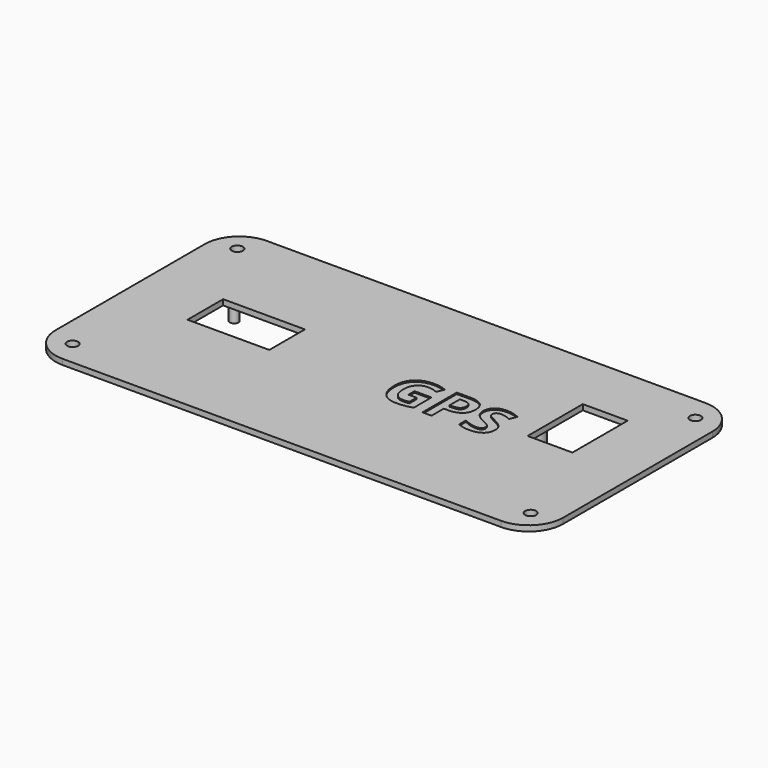
from build123d import *

# Parameters (mm, degrees)
F1_DEPTH      = 3.5
F0_W          = 147.1034944444
F0_H          = 74
F2_DEPTH      = 1.6
F3_W          = 23.7
F3_H          = 12.9
F3_W_2        = 13
F3_H_2        = 20
F4_DEPTH      = 1.601
F3_R          = 1.25
F5_DEPTH      = 5
F3_R_2        = 2.5
F6_DEPTH      = 11
F7_R          = 10
F8_R          = 1.25
F9_DEPTH      = 8
F10_R         = 1.25
F11_DEPTH     = 8
F12_R         = 1.25
F13_DEPTH     = 8
F14_R         = 1.25
F15_DEPTH     = 8
F16_R         = 1.6
F17_DEPTH     = 12.601
F19_TEXT_SIZE = 17.4003174632
F20_DEPTH     = 0.4


# Not quite as in the source:
# - Text() gives the source's letters only with a copy of the font that has no kerning and outlines rounded to 1/6400 em; it was checked with that copy


with BuildPart() as f1:
    # F0 (on Top) → F1 (new body)
    with BuildSketch(Plane.XY):
        with BuildLine():
            Line((62, 27), (-62, 27))
            Line((-62, 27), (-62, -27))
            Line((-62, -27), (62, -27))
            ThreePointArc((62, -27), (65.1034944444, 0), (62, 27))
        make_face()
        with BuildLine():
            ThreePointArc((60.7228645351, 25.4), (63.5034944444, 0), (60.7228645351, -25.4))
            Line((60.7228645351, -25.4), (-60.4, -25.4))
            Line((-60.4, -25.4), (-60.4, 25.4))
            Line((-60.4, 25.4), (60.7228645351, 25.4))
        make_face(mode=Mode.SUBTRACT)
    extrude(amount=-F1_DEPTH)


with BuildPart() as f2:
    # F0 (on Top) → F2 (new body)
    with BuildSketch(Plane.XY):
        with Locations((1.5517472222, 0)):
            Rectangle(F0_W, F0_H)
        with BuildLine():
            Line((-62, -27), (-62, 27))
            Line((-62, 27), (62, 27))
            ThreePointArc((62, 27), (65.1034944444, 0), (62, -27))
            Line((62, -27), (-62, -27))
        make_face(mode=Mode.SUBTRACT)
        with BuildLine():
            Line((62, 27), (-62, 27))
            Line((-62, 27), (-62, -27))
            Line((-62, -27), (62, -27))
            ThreePointArc((62, -27), (65.1034944444, 0), (62, 27))
        make_face()
        with BuildLine():
            ThreePointArc((60.7228645351, 25.4), (63.5034944444, 0), (60.7228645351, -25.4))
            Line((60.7228645351, -25.4), (-60.4, -25.4))
            Line((-60.4, -25.4), (-60.4, 25.4))
            Line((-60.4, 25.4), (60.7228645351, 25.4))
        make_face(mode=Mode.SUBTRACT)
        with BuildLine():
            Line((-60.4, -25.4), (60.7228645351, -25.4))
            ThreePointArc((60.7228645351, -25.4), (63.5034944444, 0), (60.7228645351, 25.4))
            Line((60.7228645351, 25.4), (-60.4, 25.4))
            Line((-60.4, 25.4), (-60.4, -25.4))
        make_face()
    extrude(amount=F2_DEPTH)

    # F3 (on face) → F4 (cut, through all)
    with BuildSketch(Plane.XY):
        with Locations((-40.0405414402, 2.075)):
            Rectangle(F3_W, F3_H)
        with Locations((50.30156672, 9.2107076198)):
            Rectangle(F3_W_2, F3_H_2)
    extrude(amount=F4_DEPTH, mode=Mode.SUBTRACT)

    # F7
    f7_edges = [f2.edges().sort_by_distance(p)[0] for p in [
        (75.103494, 37, 0.8),
        (-72, 37, 0.8),
        (-72, -37, 0.8),
        (75.103494, -37, 0.8),
    ]]
    fillet(f7_edges, radius=F7_R)

    # F16 (on face) → F17 (cut, through all)
    with BuildSketch(Plane.XY.offset(1.6)):
        with Locations((-64.8284271247, 29.8284271247)):
            Circle(F16_R)
        with Locations((67.9319215691, 29.8284271247)):
            Circle(F16_R)
        with Locations((-64.8284271247, -29.8284271247)):
            Circle(F16_R)
        with Locations((67.9319215691, -29.8284271247)):
            Circle(F16_R)
    extrude(amount=-F17_DEPTH, mode=Mode.SUBTRACT)

    # F19 (on face) → F20 (cut)
    with BuildSketch(Plane.XY.offset(1.6)):
        with Locations((3.818041645, -6.6011277959)):
            Text('GPS', F19_TEXT_SIZE, font='Open Sans', font_style=FontStyle.BOLD, text_align=(TextAlign.LEFT, TextAlign.BOTTOM))
    extrude(amount=-F20_DEPTH, mode=Mode.SUBTRACT)


with BuildPart() as f5:
    # F3 (on face) → F5 (new body)
    with BuildSketch(Plane.XY):
        with Locations((-51.1905414402, -11.65)):
            Circle(F3_R)
    extrude(amount=-F5_DEPTH)


with BuildPart() as f5b:
    # F3 (on face) → F5, piece 2 (new body)
    with BuildSketch(Plane.XY):
        with Locations((-28.8905414402, -11.65)):
            Circle(F3_R)
    extrude(amount=-F5_DEPTH)


with BuildPart() as f5c:
    # F3 (on face) → F5, piece 3 (new body)
    with BuildSketch(Plane.XY):
        with Locations((-28.8905414402, 11.65)):
            Circle(F3_R)
    extrude(amount=-F5_DEPTH)


with BuildPart() as f5d:
    # F3 (on face) → F5, piece 4 (new body)
    with BuildSketch(Plane.XY):
        with Locations((-51.1905414402, 11.65)):
            Circle(F3_R)
    extrude(amount=-F5_DEPTH)


with BuildPart() as f6:
    # F3 (on face) → F6 (new body)
    with BuildSketch(Plane.XY):
        with Locations((12.470341146, 15.25)):
            Circle(F3_R_2)
    extrude(amount=-F6_DEPTH)

    # F12 (on face) → F13 (cut)
    with BuildSketch(Plane(origin=(0, 0, -11), x_dir=(1, 0, 0), z_dir=(0, 0, -1))):
        with Locations((12.470341146, -15.25)):
            Circle(F12_R)
    extrude(amount=-F13_DEPTH, mode=Mode.SUBTRACT)


with BuildPart() as f6b:
    # F3 (on face) → F6, piece 2 (new body)
    with BuildSketch(Plane.XY):
        with Locations((33.470341146, 15.25)):
            Circle(F3_R_2)
    extrude(amount=-F6_DEPTH)

    # F14 (on face) → F15 (cut)
    with BuildSketch(Plane(origin=(0, 0, -11), x_dir=(1, 0, 0), z_dir=(0, 0, -1))):
        with Locations((33.470341146, -15.25)):
            Circle(F14_R)
    extrude(amount=-F15_DEPTH, mode=Mode.SUBTRACT)


with BuildPart() as f6c:
    # F3 (on face) → F6, piece 3 (new body)
    with BuildSketch(Plane.XY):
        with Locations((33.470341146, -15.25)):
            Circle(F3_R_2)
    extrude(amount=-F6_DEPTH)

    # F10 (on face) → F11 (cut)
    with BuildSketch(Plane(origin=(0, 0, -11), x_dir=(1, 0, 0), z_dir=(0, 0, -1))):
        with Locations((33.470341146, 15.25)):
            Circle(F10_R)
    extrude(amount=-F11_DEPTH, mode=Mode.SUBTRACT)


with BuildPart() as f6d:
    # F3 (on face) → F6, piece 4 (new body)
    with BuildSketch(Plane.XY):
        with Locations((12.470341146, -15.25)):
            Circle(F3_R_2)
    extrude(amount=-F6_DEPTH)

    # F8 (on face) → F9 (cut)
    with BuildSketch(Plane(origin=(0, 0, -11), x_dir=(1, 0, 0), z_dir=(0, 0, -1))):
        with Locations((12.470341146, 15.25)):
            Circle(F8_R)
    extrude(amount=-F9_DEPTH, mode=Mode.SUBTRACT)


solid = Compound([f1.part, f2.part, f5.part, f5b.part, f5c.part, f5d.part, f6.part, f6b.part, f6c.part, f6d.part])
